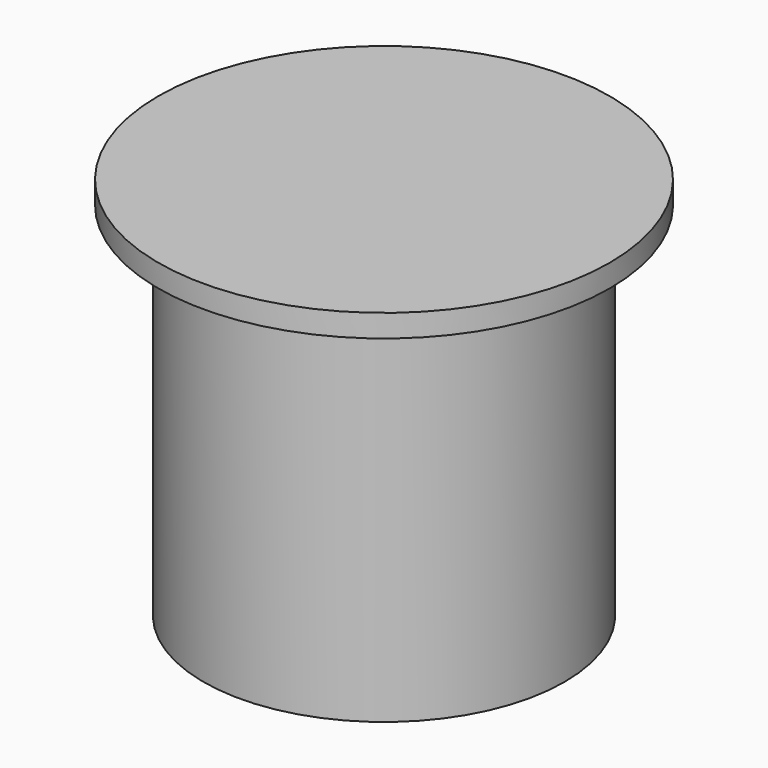
from build123d import *

# Parameters (mm, degrees)
F0_R     = 15.875
F1_DEPTH = 1.5875
F2_R     = 12.7
F3_DEPTH = 25.4


# Not quite as in the source:
# - a length typed as a fraction of an inch, garbled in the dataset ("3 / 203.2 mm" for 3/8 in), is restored


with BuildPart() as f1:
    # F0 (on Top) → F1 (new body)
    with BuildSketch(Plane.XY):
        Circle(F0_R)
    extrude(amount=F1_DEPTH)

    # F2 (on face) → F3 (join)
    with BuildSketch(Plane(origin=(0, 0, 0), x_dir=(1, 0, 0), z_dir=(0, 0, -1))):
        Circle(F2_R)
    extrude(amount=F3_DEPTH)


solid = f1.part
